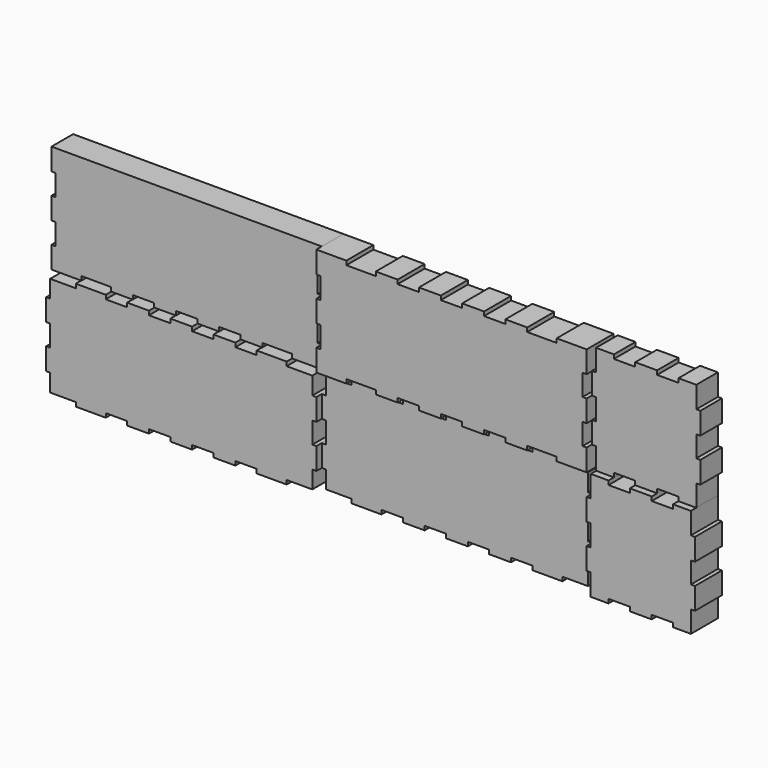
from build123d import *

# Parameters (mm, degrees)
F1_DEPTH = 25
F2_DEPTH = 20
F3_W     = 155.799987
F3_H     = 2.999999
F4_DEPTH = 20


# Not quite as in the source:
# - ends of sketch curves that miss each other by under 0.0002 mm in the source are joined


with BuildPart() as f1:
    # F0 (on Front) → F1 (new body)
    with BuildSketch(Plane.XZ):
        Polygon((176.299989, 2e-06), (163.099989, 2e-06), (163.099989, -16), (160.09999, -16), (160.09999, -32.199999), (163.099989, -32.199999), (163.099989, -47.999996), (160.09999, -47.999996), (160.09999, -64.199997), (163.099989, -64.199997), (163.099989, -80.199997), (176.299989, -80.199997), (176.299989, -77.199993), (192.099987, -77.199993), (192.099987, -80.199997), (208.299985, -80.199997), (208.299985, -77.199993), (224.099985, -77.199993), (224.099985, -80.199997), (237.299981, -80.199997), (237.299981, -64.199997), (240.299985, -64.199997), (240.299985, -47.999996), (237.299981, -47.999996), (237.299981, -32.199999), (240.299985, -32.199999), (240.299985, -16), (237.299981, -16), (237.299981, -1e-06), (224.099985, 2e-06), (224.099985, -3.000001), (208.299985, -3.000001), (208.299985, -1e-06), (192.099987, 2e-06), (192.099987, -3.000001), (176.299989, -3.000001), align=None)
    extrude(amount=F1_DEPTH)


with BuildPart() as f1b:
    # F0 (on Front) → F1, piece 2 (new body)
    with BuildSketch(Plane.XZ):
        Polygon((-218.099985, 2e-06), (-218.299986, 2e-06), (-218.299986, -3.000001), (-237.299985, -3.000001), (-237.299985, -16), (-240.299985, -16), (-240.299985, -32.199999), (-237.299985, -32.199999), (-237.299985, -47.999996), (-240.299985, -47.999996), (-240.299985, -64.199997), (-237.299985, -64.199997), (-237.299985, -77.199993), (-218.299986, -77.199993), (-218.299986, -80.199997), (-196.099987, -80.199997), (-196.099987, -77.199993), (-180.299987, -77.199993), (-180.299987, -80.199997), (-164.099991, -80.199997), (-164.099991, -77.199993), (-148.299988, -77.199993), (-148.299988, -80.199997), (-132.099992, -80.199997), (-132.099992, -77.199993), (-116.299988, -77.199993), (-116.299988, -80.199997), (-100.099992, -80.199997), (-100.099992, -77.199993), (-84.299997, -77.199993), (-84.299997, -80.199997), (-62.099994, -80.199997), (-62.099994, -77.199993), (-43.099999, -77.199993), (-43.099999, -64.199997), (-40.099995, -64.199997), (-40.099995, -47.999996), (-43.099999, -47.999996), (-43.099999, -32.199999), (-40.099995, -32.199999), (-40.099995, -16), (-43.099999, -16), (-43.099999, -3.000001), (-62.099994, -3.000001), (-62.099994, -1e-06), (-62.299998, 2e-06), (-84.099992, -1e-06), (-84.299997, 2e-06), (-84.299997, -3.000001), (-100.099992, -3.000001), (-100.099992, -1e-06), (-100.299997, 2e-06), (-116.099992, -1e-06), (-116.299988, 2e-06), (-116.299988, -3.000001), (-132.099992, -3.000001), (-132.099992, -1e-06), (-132.299988, 2e-06), (-148.099992, -1e-06), (-148.299988, 2e-06), (-148.299988, -3.000001), (-164.099991, -3.000001), (-164.099991, -1e-06), (-164.299988, 2e-06), (-180.099987, -1e-06), (-180.299987, 2e-06), (-180.299987, -3.000001), (-196.099987, -3.000001), (-196.099987, -1e-06), (-196.299987, 2e-06), align=None)
    extrude(amount=F1_DEPTH)


with BuildPart() as f1c:
    # F0 (on Front) → F1, piece 3 (new body)
    with BuildSketch(Plane.XZ):
        Polygon((-17.900001, 80.199997), (-40.1, 80.199997), (-40.099995, 63.999998), (-37.100001, 63.999998), (-37.100001, 48.2), (-40.1, 48.2), (-40.099995, 32.000002), (-37.100001, 32.000002), (-37.100001, 16.200002), (-40.1, 16.200002), (-40.099995, 2e-06), (-18.100002, 2e-06), (-17.900001, 2e-06), (-17.900001, 3.000006), (3.899997, 3.000006), (3.899997, 2e-06), (4.099998, 2e-06), (19.899997, 2e-06), (20.099998, 2e-06), (20.099998, 3.000006), (35.899997, 3.000006), (35.899997, 2e-06), (36.099993, 2e-06), (51.899997, 2e-06), (52.099993, 2e-06), (52.099993, 3.000006), (67.899996, 3.000006), (67.899996, 2e-06), (68.099993, 2e-06), (83.899996, 2e-06), (84.099993, 2e-06), (84.099993, 3.000006), (99.899988, 3.000006), (99.899988, 2e-06), (100.099992, 2e-06), (115.899987, 2e-06), (116.099992, 2e-06), (116.099992, 3.000006), (137.899986, 3.000006), (137.899986, 2e-06), (138.099991, 2e-06), (160.09999, 2e-06), (160.09999, 16.000002), (160.09999, 16.200002), (157.099986, 16.200002), (157.099986, 32.000002), (160.09999, 32.000002), (160.09999, 32.200002), (160.09999, 47.999999), (160.09999, 48.2), (157.099986, 48.2), (157.099986, 63.999998), (160.09999, 63.999998), (160.09999, 64.199999), (160.09999, 80.199997), (137.899986, 80.199997), (137.899986, 77.199998), (116.099992, 77.199998), (116.099992, 80.199997), (99.899988, 80.199997), (99.899988, 77.199998), (84.099993, 77.199998), (84.099993, 80.199997), (67.899996, 80.199997), (67.899996, 77.199998), (52.099993, 77.199998), (52.099993, 80.199997), (35.899997, 80.199997), (35.899997, 77.199998), (20.099998, 77.199998), (20.099998, 80.199997), (3.899997, 80.199997), (3.899997, 77.199998), (-17.900001, 77.199998), align=None)
    extrude(amount=F1_DEPTH)


with BuildPart() as f2:
    # F0 (on Front) → F2 (new body)
    with BuildSketch(Plane.XZ):
        Polygon((-218.099985, 80.199997), (-240.299985, 80.199997), (-240.299985, 63.999998), (-237.299985, 63.999998), (-237.299985, 48.2), (-240.299985, 48.2), (-240.299985, 32.000002), (-237.299985, 32.000002), (-237.299985, 16.200002), (-240.299985, 16.200002), (-240.299985, 2e-06), (-218.299986, 2e-06), (-218.099985, 2e-06), (-218.099985, 3.000006), (-196.299987, 3.000006), (-196.299987, 2e-06), (-196.099987, 2e-06), (-180.299987, 2e-06), (-180.099987, 2e-06), (-180.099987, 3.000006), (-164.299988, 3.000006), (-164.299988, 2e-06), (-164.099991, 2e-06), (-148.299988, 2e-06), (-148.099992, 2e-06), (-148.099992, 3.000006), (-132.299988, 3.000006), (-132.299988, 2e-06), (-132.099992, 2e-06), (-116.299988, 2e-06), (-116.099992, 2e-06), (-116.099992, 3.000006), (-100.299997, 3.000006), (-100.299997, 2e-06), (-100.099992, 2e-06), (-84.299997, 2e-06), (-84.099992, 2e-06), (-84.099992, 3.000006), (-62.299998, 3.000006), (-62.299998, 2e-06), (-62.099994, 2e-06), (-40.099995, 2e-06), (-40.099995, 16.200002), (-43.099999, 16.200002), (-43.099999, 32.000002), (-40.099995, 32.000002), (-40.099995, 48.2), (-43.099999, 48.2), (-43.099999, 63.999998), (-40.099995, 63.999998), (-40.099995, 80.199997), (-62.299998, 80.199997), (-62.299998, 77.199998), (-84.099992, 77.199998), (-84.099992, 80.199997), (-100.299997, 80.199997), (-100.299997, 77.199998), (-116.099992, 77.199998), (-116.099992, 80.199997), (-132.299988, 80.199997), (-132.299988, 77.199998), (-148.099992, 77.199998), (-148.099992, 80.199997), (-164.299988, 80.199997), (-164.299988, 77.199998), (-180.099987, 77.199998), (-180.099987, 80.199997), (-196.299987, 80.199997), (-196.299987, 77.199998), (-218.099985, 77.199998), align=None)
    extrude(amount=F2_DEPTH)

    # F3 (on face) → F4 (join)
    with BuildSketch(Plane.XZ.offset(20)):
        with Locations((-140.1999915, 78.6999975)):
            Rectangle(F3_W, F3_H)
    extrude(amount=-F4_DEPTH)


with BuildPart() as f2b:
    # F0 (on Front) → F2, piece 2 (new body)
    with BuildSketch(Plane.XZ):
        Polygon((-17.900001, 2e-06), (-18.100002, 2e-06), (-18.100002, -3.000001), (-37.100001, -3.000001), (-37.100001, -16), (-40.1, -16), (-40.099995, -32.199999), (-37.100001, -32.199999), (-37.100001, -47.999996), (-40.1, -47.999996), (-40.099995, -64.199997), (-37.100001, -64.199997), (-37.100001, -77.199993), (-18.100002, -77.199993), (-18.100002, -80.199997), (4.099998, -80.199997), (4.099998, -77.199993), (19.899997, -77.199993), (19.899997, -80.199997), (36.099993, -80.199997), (36.099993, -77.199993), (51.899997, -77.199993), (51.899997, -80.199997), (68.099993, -80.199997), (68.099993, -77.199993), (83.899996, -77.199993), (83.899996, -80.199997), (100.099992, -80.199997), (100.099992, -77.199993), (115.899987, -77.199993), (115.899987, -80.199997), (138.099991, -80.199997), (138.099991, -77.199993), (157.099986, -77.199993), (157.099986, -64.199997), (160.09999, -64.199997), (160.09999, -47.999996), (157.099986, -47.999996), (157.099986, -32.199999), (160.09999, -32.199999), (160.09999, -16), (157.099986, -16), (157.099986, -3.000001), (138.099991, -3.000001), (138.099991, -1e-06), (137.899986, 2e-06), (116.099992, -1e-06), (115.899987, 2e-06), (115.899987, -3.000001), (100.099992, -3.000001), (100.099992, -1e-06), (99.899988, 2e-06), (84.099993, -1e-06), (83.899996, 2e-06), (83.899996, -3.000001), (68.099993, -3.000001), (68.099993, -1e-06), (67.899996, 2e-06), (52.099993, -1e-06), (51.899997, 2e-06), (51.899997, -3.000001), (36.099993, -3.000001), (36.099993, -1e-06), (35.899997, 2e-06), (20.099998, -1e-06), (19.899997, 2e-06), (19.899997, -3.000001), (4.099998, -3.000001), (4.099998, -1e-06), (3.899997, 2e-06), align=None)
    extrude(amount=F2_DEPTH)


with BuildPart() as f2c:
    # F0 (on Front) → F2, piece 3 (new body)
    with BuildSketch(Plane.XZ):
        Polygon((163.099989, 64.199999), (160.09999, 64.199999), (160.09999, 63.999998), (160.09999, 48.2), (160.09999, 47.999999), (163.099989, 47.999999), (163.099989, 32.200002), (160.09999, 32.200002), (160.09999, 32.000002), (160.09999, 16.200002), (160.09999, 16.000002), (163.099989, 16.000002), (163.099989, 2e-06), (176.299989, 2e-06), (176.299989, 3.000006), (192.099987, 3.000006), (192.099987, 2e-06), (208.299985, 2e-06), (208.299985, 3.000006), (224.099985, 3.000006), (224.099985, 2e-06), (237.299981, 2e-06), (237.299981, 16.000002), (240.299985, 16.000002), (240.299985, 32.200002), (237.299981, 32.200002), (237.299981, 47.999999), (240.299985, 47.999999), (240.299985, 64.199999), (237.299981, 64.199999), (237.299981, 80.199997), (224.099985, 80.199997), (224.099985, 77.199998), (208.299985, 77.199998), (208.299985, 80.199997), (192.099987, 80.199997), (192.099987, 77.199998), (176.299989, 77.199998), (176.299989, 80.199997), (163.099989, 80.199997), align=None)
    extrude(amount=F2_DEPTH)


solid = Compound([f1.part, f1b.part, f1c.part, f2.part, f2b.part, f2c.part])
